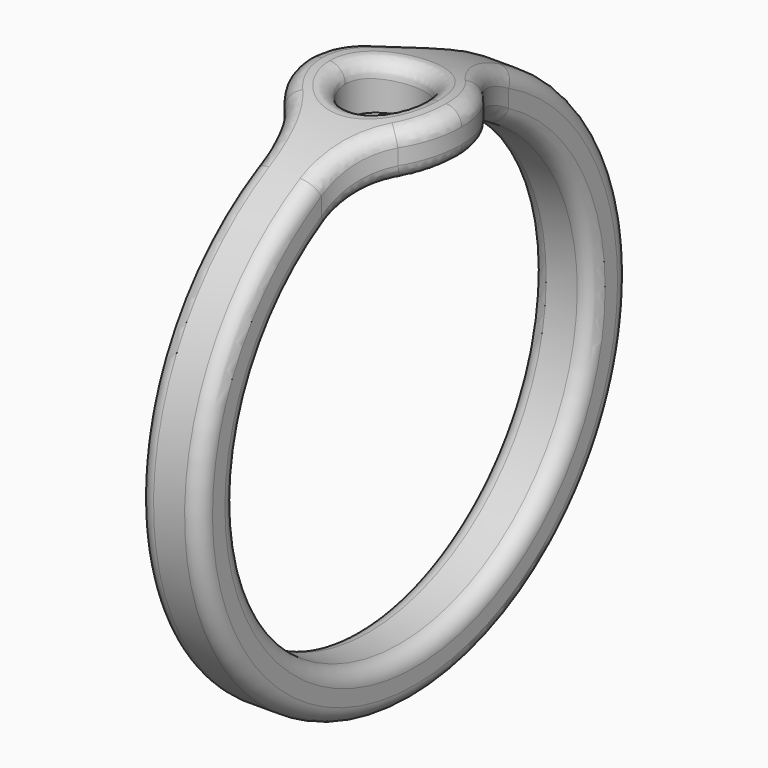
from build123d import *

# Parameters (mm, degrees)
F0_W     = 5
F0_H     = 1.5
F2_R     = 1.25
F3_DEPTH = 8.6625
F4_W     = 3.5563625172
F4_H     = 19.9871556833
F4_W_2   = 2.223615
F5_DEPTH = 25
F6_R     = 0.5
F7_R     = 0.5


# Not quite as in the source:
# - a feature names something its author has since deleted; it is built from what else it names


with BuildPart() as f1:
    # F0 (on Front) → F1 (revolve)
    with BuildSketch(Plane.XZ):
        with Locations((0, 7.9115)):
            Rectangle(F0_W, F0_H)
    revolve(axis=Axis((1.2177848257, 0, 0), (1, 0, 0)))

    # F2 (on Top) → F3 (cut, through all)
    with BuildSketch(Plane.XY):
        with BuildLine():
            Line((-1, 3.7749172176), (-1, 13.7922661379))
            Line((-1, 13.7922661379), (-4.3010441586, 13.7922661379))
            Line((-4.3010441586, 13.7922661379), (-4.3010441586, -10.5645237491))
            Line((-4.3010441586, -10.5645237491), (-1, -10.5645237491))
            Line((-1, -10.5645237491), (-1, -3.7749172176))
            ThreePointArc((-1, -3.7749172176), (-1.2120388681, -2.6670937988), (-1.8181818182, -1.7158714626))
            ThreePointArc((-1.8181818182, -1.7158714626), (-2.5, 0), (-1.8181818182, 1.7158714626))
            ThreePointArc((-1.8181818182, 1.7158714626), (-1.2120388681, 2.6670937988), (-1, 3.7749172176))
        make_face()
        with BuildLine():
            ThreePointArc((1.8181818182, 1.7158714626), (2.5, 0), (1.8181818182, -1.7158714626))
            ThreePointArc((1.8181818182, -1.7158714626), (1.2120388681, -2.6670937988), (1, -3.7749172176))
            Line((1, -3.7749172176), (1, -10.5645237491))
            Line((1, -10.5645237491), (5.0637214445, -10.5645237491))
            Line((5.0637214445, -10.5645237491), (5.0637214445, 13.7922661379))
            Line((5.0637214445, 13.7922661379), (1, 13.7922661379))
            Line((1, 13.7922661379), (1, 3.7749172176))
            ThreePointArc((1, 3.7749172176), (1.2120388681, 2.6670937988), (1.8181818182, 1.7158714626))
        make_face()
        Circle(F2_R)
    extrude(amount=F3_DEPTH, mode=Mode.SUBTRACT)

    # F4 (on Top) → F5 (cut)
    with BuildSketch(Plane.XY):
        with Locations((-2.7781812586, 0.4311273806)):
            Rectangle(F4_W, F4_H)
        with Locations((2.1118075, 0.4311273806)):
            Rectangle(F4_W_2, F4_H)
    extrude(amount=-F5_DEPTH, mode=Mode.SUBTRACT)

    # F6
    f6_edges = [f1.edges().sort_by_distance(p)[0] for p in [
        (1, 0, -7.1615),
        (-1, 0, -7.1615),
    ]]
    fillet(f6_edges, radius=F6_R)

    # F7
    f7_edges = [f1.edges().sort_by_distance(p)[0] for p in [
        (0, -1.25, 8.570827),
        (0, 1.25, 8.570827),
        (-2.304784, -0.968489, 8.607184),
        (-2.305806, 0.966053, 8.607457),
        (-1.214167, -2.661752, 8.24237),
        (1.214166, 2.661757, 8.242368),
        (2.304784, 0.968489, 8.607184),
        (-1.214166, 2.661757, 8.242368),
        (-1, 0, -8.6615),
        (2.305806, -0.966053, 8.607457),
        (1.214167, -2.661752, 8.24237),
        (1, 0, -8.6615),
    ]]
    fillet(f7_edges, radius=F7_R)


solid = f1.part
